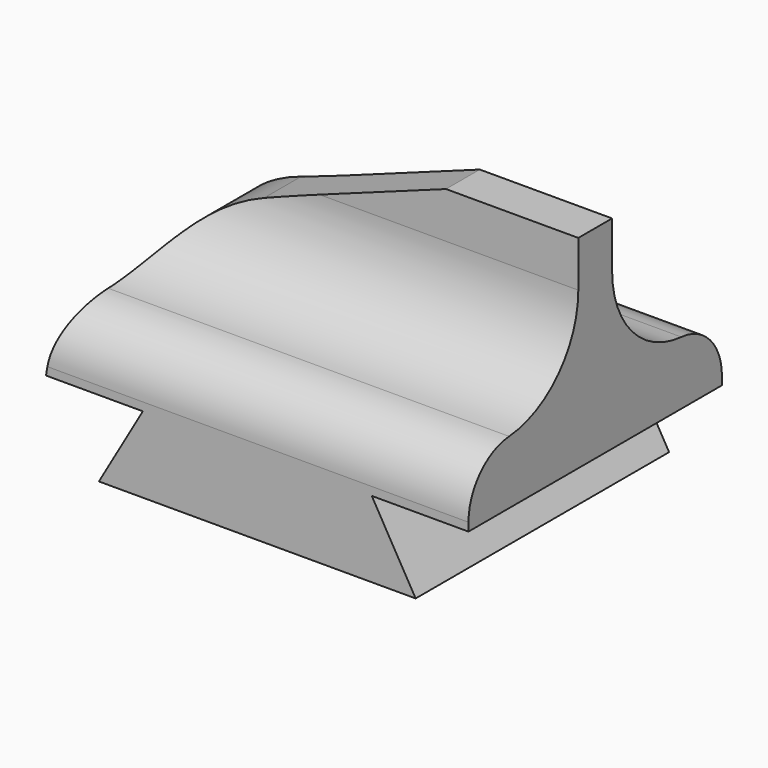
from build123d import *

# Parameters (mm, degrees)
F0_W         = 9.525
F0_H         = 9.525
F1_DEPTH     = 2.286
F2_T1_DEPTH  = 21.3619144247
F3_W         = 2.9083
F3_H         = 9.525
F3_W_2       = 6.8834
F4_DEPTH     = 1.905
F5_R         = 1.6556676611
F6_W         = 12.7
F6_H         = 1.27
F7_DEPTH     = 4.191
F8_SIZE2     = 8.7232408068
F8_SIZE      = 3.175
F9_T4_DEPTH  = 12.7
F9_T9_DEPTH  = 12.7
F10_T1_DEPTH = 20.1155023365


# Not quite as in the source:
# - a fillet or chamfer that OpenCascade refuses, or shapes differently, is made with other operations: its cross-section is extruded or revolved along the edge and cut away or added


with BuildPart() as f1:
    # F0 (on Top) → F1 (new body)
    with BuildSketch(Plane.XY):
        Rectangle(F0_W, F0_H)
    extrude(amount=F1_DEPTH)

    # F2: chamfer of 1.3208 x 2.2876927066 on 2 edges, made by hand

    # F2_s2 → F2_t1 (cut)
    with BuildSketch(Plane.XZ.offset(-10.6809572123)):
        Polygon((-4.7625, -0.0016927066), (-3.4417, 2.286), (-4.7625, 2.286), align=None)
        Polygon((4.7625, -0.0016927066), (3.4417, 2.286), (4.7625, 2.286), align=None)
    extrude(amount=F2_T1_DEPTH, mode=Mode.SUBTRACT)

    # F3 (on face) → F4 (join)
    with BuildSketch(Plane.XY.offset(2.286)):
        with Locations((4.89585, 0)):
            Rectangle(F3_W, F3_H)
        Rectangle(F3_W_2, F3_H)
        with Locations((-4.89585, 0)):
            Rectangle(F3_W, F3_H)
    extrude(amount=F4_DEPTH)

    # F5
    f5_edges = [f1.edges().sort_by_distance(p)[0] for p in [
        (0, 4.7625, 4.191),
        (0, -4.7625, 4.191),
    ]]
    fillet(f5_edges, radius=F5_R)

    # F6 (on face) → F7 (join)
    with BuildSketch(Plane.XY.offset(4.191)):
        Rectangle(F6_W, F6_H)
    extrude(amount=F7_DEPTH)

    # F8
    f8_edges = [f1.edges().sort_by_distance(p)[0] for p in [
        (-6.35, 0, 8.382),
    ]]
    f8_side = f1.faces().sort_by_distance((-6.35, 0, 3.935532))[0]
    chamfer(f8_edges, length=F8_SIZE, length2=F8_SIZE2, reference=f8_side)

    # F9: fillet of radius 2.8207671263 on 2 edges, made by hand


with BuildPart() as f9_tool2:
    # F9_s3 → F9_t4 (new body)
    with BuildSketch(Plane.YZ.offset(-6.35)):
        with BuildLine():
            ThreePointArc((-0.635, 6.9981468006), (-1.3849039981, 5.0828783899), (-3.235890411, 4.1859623453))
            Line((-3.235890411, 4.1859623453), (-3.2139027394, 3.9047438998))
            ThreePointArc((-3.2139027394, 3.9047438998), (-3.1068323389, 3.9089232874), (-0.635, 3.9089232874))
            Line((-0.635, 3.9089232874), (-0.3529232874, 4.191))
            Line((-0.3529232874, 4.191), (-0.3529232874, 6.9981468006))
            Line((-0.3529232874, 6.9981468006), (-0.635, 6.9981468006))
        make_face()
    extrude(amount=F9_T4_DEPTH)

    split(bisect_by=Plane(origin=(-2.4163064349, 0, 6.6387473684), x_dir=(0, 1, 0), z_dir=(0.3420201433, 0, -0.9396926208)), keep=Keep.TOP)


with BuildPart() as f1_1:
    add(f1.part)

    # F9_t1: union F9_tool2
    add(f9_tool2.part)


with BuildPart() as f9_tool7:
    # F9_s8 → F9_t9 (new body)
    with BuildSketch(Plane.YZ.offset(6.35)):
        with BuildLine():
            ThreePointArc((0.635, 6.9981468006), (1.3849039981, 5.0828783899), (3.235890411, 4.1859623453))
            Line((3.235890411, 4.1859623453), (3.2139027394, 3.9047438998))
            ThreePointArc((3.2139027394, 3.9047438998), (3.1068323389, 3.9089232874), (0.635, 3.9089232874))
            Line((0.635, 3.9089232874), (0.3529232874, 4.191))
            Line((0.3529232874, 4.191), (0.3529232874, 6.9981468006))
            Line((0.3529232874, 6.9981468006), (0.635, 6.9981468006))
        make_face()
    extrude(amount=-F9_T9_DEPTH)

    split(bisect_by=Plane(origin=(-2.4163064349, 0, 6.6387473684), x_dir=(0, 1, 0), z_dir=(0.3420201433, 0, -0.9396926208)), keep=Keep.TOP)


with BuildPart() as f1_2:
    add(f1_1.part)

    # F9_t6: union F9_tool7
    add(f9_tool7.part)

    # F10: fillet of radius 5.08 on 1 edges, made by hand

    # F10_s2 → F10_t1 (cut)
    with BuildSketch(Plane.XZ.offset(-10.0577511683)):
        with BuildLine():
            ThreePointArc((-6.35, 2.286), (-5.2774477357, 4.8097508006), (-3.0493882968, 6.4083244148))
            Line((-3.0493882968, 6.4083244148), (-3.0841375434, 6.5037971851))
            Line((-3.0841375434, 6.5037971851), (-6.3847492466, 5.3024727703))
            Line((-6.3847492466, 5.3024727703), (-6.4516, 5.207))
            ThreePointArc((-6.4516, 5.207), (-6.4516, 3.7465), (-6.4507614806, 2.299026282))
            Line((-6.4507614806, 2.299026282), (-6.35, 2.286))
        make_face()
    extrude(amount=F10_T1_DEPTH, mode=Mode.SUBTRACT)


solid = f1_2.part
